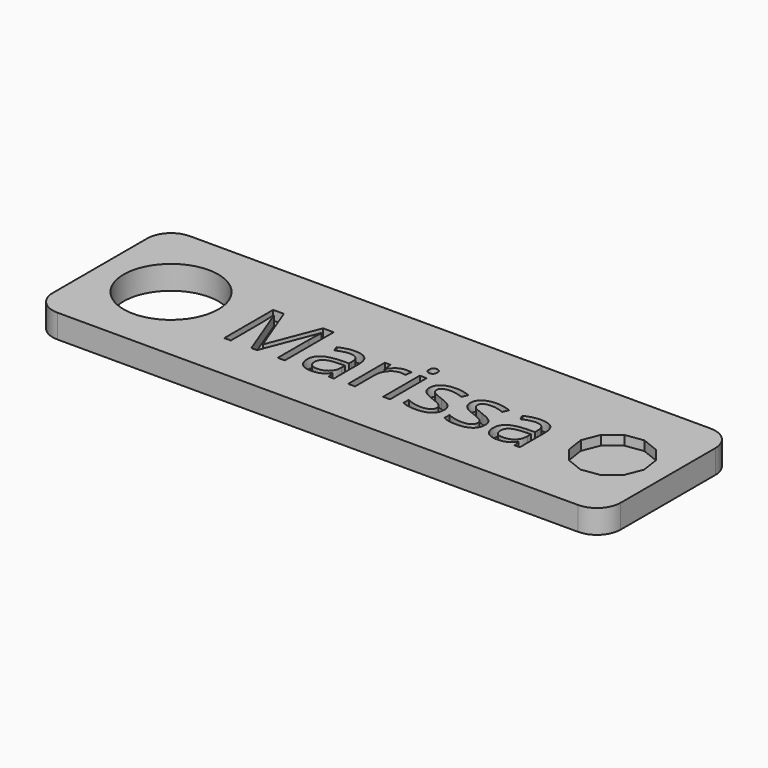
from build123d import *

# Parameters (mm, degrees)
F0_W         = 120
F0_H         = 35
F0_R         = 10
F1_DEPTH     = 5
F2_R         = 5
F3_TEXT_SIZE = 18.0921064586
F4_DEPTH     = 4.7
F5_DEPTH     = 2


# Not quite as in the source:
# - Text() gives the source's letters only with a copy of the font that has no kerning and outlines rounded to 1/6400 em; it was checked with that copy


with BuildPart() as f1:
    # F0 (on Top) → F1 (new body)
    with BuildSketch(Plane.XY):
        Rectangle(F0_W, F0_H)
        with Locations((-45, 0)):
            Circle(F0_R, mode=Mode.SUBTRACT)
    extrude(amount=F1_DEPTH)

    # F2
    f2_edges = [f1.edges().sort_by_distance(p)[0] for p in [
        (-60, -17.5, 2.5),
        (60, -17.5, 2.5),
        (60, 17.5, 2.5),
        (-60, 17.5, 2.5),
    ]]
    fillet(f2_edges, radius=F2_R)

    # F3 (on face) → F4 (cut)
    with BuildSketch(Plane.XY.offset(5)):
        Polygon((51.1901535741, -6.8149062957), (54.2045823583, -4.4350950827), (55.6252486568, -0.8669037239), (55.0714860822, 2.9335737875), (52.6916748692, 5.9480025717), (49.1234835105, 7.3686688702), (45.323005999, 6.8149062957), (42.3085772148, 4.4350950827), (40.8879109163, 0.8669037239), (41.4416734909, -2.9335737875), (43.8214847039, -5.9480025717), (47.3896760626, -7.3686688702), align=None)
        with Locations((-29.6052638441, -7.401315961)):
            Text('Marissa', F3_TEXT_SIZE, font='Open Sans', text_align=(TextAlign.LEFT, TextAlign.BOTTOM))
    extrude(amount=F4_DEPTH, mode=Mode.SUBTRACT)

    # F3 (on face) → F5 (cut)
    with BuildSketch(Plane.XY.offset(5)):
        Polygon((51.1901535741, -6.8149062957), (54.2045823583, -4.4350950827), (55.6252486568, -0.8669037239), (55.0714860822, 2.9335737875), (52.6916748692, 5.9480025717), (49.1234835105, 7.3686688702), (45.323005999, 6.8149062957), (42.3085772148, 4.4350950827), (40.8879109163, 0.8669037239), (41.4416734909, -2.9335737875), (43.8214847039, -5.9480025717), (47.3896760626, -7.3686688702), align=None)
        with Locations((-29.6052638441, -7.401315961)):
            Text('Marissa', F3_TEXT_SIZE, font='Open Sans', text_align=(TextAlign.LEFT, TextAlign.BOTTOM))
    extrude(amount=-F5_DEPTH, mode=Mode.SUBTRACT)


solid = f1.part
